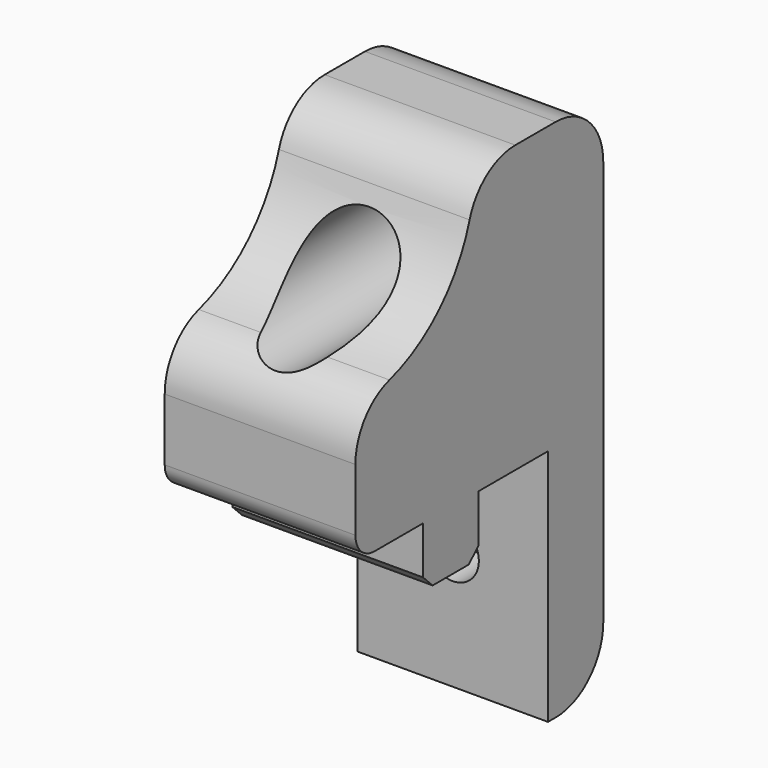
from build123d import *

# Parameters (mm, degrees)
F0_W           = 16
F0_H           = 24
F1_DEPTH       = 13
F2_W           = 16
F2_H           = 5.8
F3_DEPTH       = 5
F4_DEPTH       = 20
F5_R           = 4.05
F6_DEPTH       = 26.001
F8_D           = 4.4
F8_CBORE_D     = 8.25
F8_CBORE_DEPTH = 2
F9_SIZE        = 1
F11_DEPTH      = 16.001
F12_T1_DEPTH   = 27.2312288127
F12_T3_DEPTH   = 27.2312288127
F12_T5_DEPTH   = 41
F12_T7_DEPTH   = 37.3525491562
F13_R          = 2


# Not quite as in the source:
# - a fillet or chamfer that OpenCascade refuses, or shapes differently, is made with other operations: its cross-section is extruded or revolved along the edge and cut away or added
# - a feature names something its author has since deleted; it is built from what else it names


with BuildPart() as f1:
    # F0 (on Front) → F1 (new body, symmetric)
    with BuildSketch(Plane.XZ):
        Rectangle(F0_W, F0_H)
    extrude(amount=F1_DEPTH, both=True)

    # F2 (on face) → F3 (join)
    with BuildSketch(Plane(origin=(0, 0, -12), x_dir=(1, 0, 0), z_dir=(0, 0, -1))):
        with Locations((0, 3)):
            Rectangle(F2_W, F2_H)
    extrude(amount=F3_DEPTH)

    # F2 (on face) → F4 (join)
    with BuildSketch(Plane(origin=(0, 0, -12), x_dir=(1, 0, 0), z_dir=(0, 0, -1))):
        with Locations((0, -10.1)):
            Rectangle(F2_W, F2_H)
    extrude(amount=F4_DEPTH)

    # F5 (on face) → F6 (cut, through all)
    with BuildSketch(Plane.XZ.offset(13)):
        with Locations((0, 2.95)):
            Circle(F5_R)
    extrude(amount=-F6_DEPTH, mode=Mode.SUBTRACT)

    # F8 (through all)
    with Locations(Plane(origin=(0, 13, 0), x_dir=(-1, 0, 0), z_dir=(0, 1, 0))):
        with Locations((0, -22)):
            CounterBoreHole(F8_D / 2, F8_CBORE_D / 2, F8_CBORE_DEPTH)

    # F9
    f9_edges = [f1.edges().sort_by_distance(p)[0] for p in [
        (0, -5.9, -17),
        (0, -0.1, -17),
    ]]
    chamfer(f9_edges, length=F9_SIZE)

    # F10 (on face) → F11 (cut, through all)
    with BuildSketch(Plane.YZ.offset(8)):
        with BuildLine():
            Line((-13, 12), (-0.5, 12))
            ThreePointArc((-0.5, 12), (-21.8388347648, 20.8388347648), (-13, -0.5))
            Line((-13, -0.5), (-13, 12))
        make_face()
        with BuildLine():
            ThreePointArc((-13, -0.5), (-4.1611652352, 3.1611652352), (-0.5, 12))
            Line((-0.5, 12), (-13, 12))
            Line((-13, 12), (-13, -0.5))
        make_face()
    extrude(amount=-F11_DEPTH, mode=Mode.SUBTRACT)

    # F12: fillet of radius 5 on 5 edges, made by hand

    # F12_s2 → F12_t1 (cut)
    with BuildSketch(Plane.YZ.offset(-8.5549542346)):
        with BuildLine():
            ThreePointArc((-9.4285714286, 0.0210644063), (-12.0089186287, -1.7824383079), (-13, -4.7705098312))
            Line((-13, -4.7705098312), (-13, -0.5))
            ThreePointArc((-13, -0.5), (-11.1953802231, -0.369047961), (-9.4285714286, 0.0210644063))
        make_face()
    extrude(amount=F12_T1_DEPTH, mode=Mode.SUBTRACT)

    # F12_s4 → F12_t3 (cut)
    with BuildSketch(Plane.YZ.offset(-18.6762745781)):
        with BuildLine():
            ThreePointArc((-9.4285714286, 0.0210644063), (-12.0089186287, -1.7824383079), (-13, -4.7705098312))
            Line((-13, -4.7705098312), (-13, -0.5))
            ThreePointArc((-13, -0.5), (-11.1953802231, -0.369047961), (-9.4285714286, 0.0210644063))
        make_face()
    extrude(amount=F12_T3_DEPTH, mode=Mode.SUBTRACT)

    # F12_s6 → F12_t5 (cut)
    with BuildSketch(Plane.YZ.offset(-20.5)):
        with BuildLine():
            ThreePointArc((8, -32), (11.5355339059, -30.5355339059), (13, -27))
            Line((13, -27), (13, -32))
            Line((13, -32), (8, -32))
        make_face()
        with BuildLine():
            ThreePointArc((13, 7), (11.5355339059, 10.5355339059), (8, 12))
            Line((8, 12), (13, 12))
            Line((13, 12), (13, 7))
        make_face()
    extrude(amount=F12_T5_DEPTH, mode=Mode.SUBTRACT)

    # F12_s8 → F12_t7 (cut)
    with BuildSketch(Plane.YZ.offset(-18.6762745781)):
        with BuildLine():
            ThreePointArc((3.7705098312, 12), (0.7824383079, 11.0089186287), (-1.0210644063, 8.4285714286))
            ThreePointArc((-1.0210644063, 8.4285714286), (-0.630952039, 10.1953802231), (-0.5, 12))
            Line((-0.5, 12), (3.7705098312, 12))
        make_face()
    extrude(amount=F12_T7_DEPTH, mode=Mode.SUBTRACT)

    # F13
    f13_edges = [f1.edges().sort_by_distance(p)[0] for p in [
        (0, -13, -12),
    ]]
    fillet(f13_edges, radius=F13_R)


solid = f1.part
